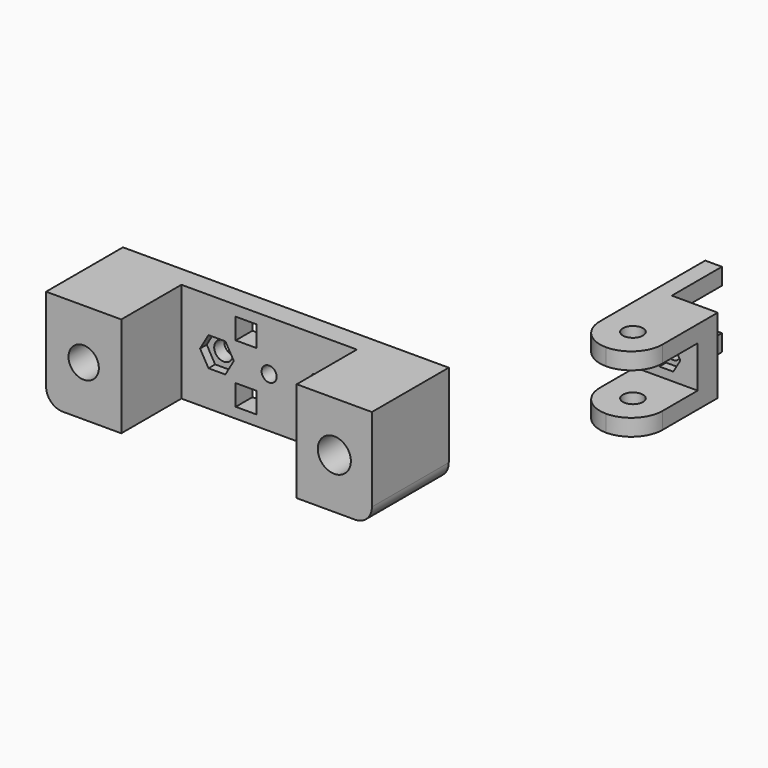
from build123d import *

# Parameters (mm, degrees)
F0_W      = 78
F0_H      = 24
F1_DEPTH  = 5
F2_R      = 2.25
F3_DEPTH  = 25
F4_DEPTH  = 2
F5_W      = 5
F5_H      = 5
F6_DEPTH  = 25
F7_W      = 18
F7_H      = 24
F8_DEPTH  = 18
F9_R      = 3.6317619329
F9_R_2    = 3.9628945372
F10_DEPTH = 30
F11_R     = 4
F2_R_2    = 1.8
F12_DEPTH = 25
F14_DEPTH = 18
F15_W     = 15
F15_H     = 10
F16_DEPTH = 25
F17_W     = 18
F17_H     = 10
F18_DEPTH = 25
F19_R     = 2.4
F20_DEPTH = 25
F21_R     = 7.49999
F22_R     = 1.8
F23_DEPTH = 25
F24_DEPTH = 2


# Not quite as in the source:
# - a fillet or chamfer is up to 0.001 mm smaller than in the source, because OpenCascade refuses the exact size


with BuildPart() as f1:
    # F0 (on Front) → F1 (new body)
    with BuildSketch(Plane.XZ):
        with Locations((-10.7673791122, -2.1172289916)):
            Rectangle(F0_W, F0_H)
    extrude(amount=F1_DEPTH)

    # F2 (on face) → F3 (cut)
    with BuildSketch(Plane.XZ.offset(5)):
        with Locations((-23.2673791122, -2.1172289916)):
            Circle(F2_R)
        with Locations((1.7326208878, -2.1172289916)):
            Circle(F2_R)
    extrude(amount=-F3_DEPTH, mode=Mode.SUBTRACT)

    # F2 (on face) → F4 (cut)
    with BuildSketch(Plane.XZ.offset(5)):
        Polygon((-21.24665317, 1.3827710084), (-25.2881050544, 1.3827710084), (-27.3088309965, -2.1172289916), (-25.2881050544, -5.6172289916), (-21.24665317, -5.6172289916), (-19.2259272279, -2.1172289916), align=None)
        with Locations((-23.2673791122, -2.1172289916)):
            Circle(F2_R, mode=Mode.SUBTRACT)
        Polygon((3.75334683, 1.3827710084), (-0.2881050544, 1.3827710084), (-2.3088309965, -2.1172289916), (-0.2881050544, -5.6172289916), (3.75334683, -5.6172289916), (5.7740727721, -2.1172289916), align=None)
        with Locations((1.7326208878, -2.1172289916)):
            Circle(F2_R, mode=Mode.SUBTRACT)
    extrude(amount=-F4_DEPTH, mode=Mode.SUBTRACT)

    # F5 (on face) → F6 (cut)
    with BuildSketch(Plane.XZ.offset(5)):
        with Locations((-16.2673791122, -9.1172289916)):
            Rectangle(F5_W, F5_H)
        with Locations((-16.2673791122, 4.8827710084)):
            Rectangle(F5_W, F5_H)
    extrude(amount=-F6_DEPTH, mode=Mode.SUBTRACT)

    # F7 (on face) → F8 (join)
    with BuildSketch(Plane.XZ.offset(5)):
        with Locations((-40.7673791122, -2.1172289916)):
            Rectangle(F7_W, F7_H)
        with Locations((19.2326208878, -2.1172289916)):
            Rectangle(F7_W, F7_H)
    extrude(amount=F8_DEPTH)

    # F9 (on face) → F10 (cut, symmetric)
    with BuildSketch(Plane.XZ.offset(5)):
        with Locations((-40.7673791122, -2.1172289916)):
            Circle(F9_R)
        with Locations((19.2326208878, -2.1172289916)):
            Circle(F9_R_2)
    extrude(amount=F10_DEPTH, both=True, mode=Mode.SUBTRACT)

    # F11
    f11_edges = [f1.edges().sort_by_distance(p)[0] for p in [
        (-49.767379, -11.5, -14.117229),
        (28.232621, -11.5, -14.117229),
    ]]
    fillet(f11_edges, radius=F11_R)

    # F2 (on face) → F12 (cut)
    with BuildSketch(Plane.XZ.offset(5)):
        with Locations((-10.7673791122, -2.1172289916)):
            Circle(F2_R_2)
    extrude(amount=-F12_DEPTH, mode=Mode.SUBTRACT)


with BuildPart() as f14:
    # F13 (on Top) → F14 (new body)
    with BuildSketch(Plane.XY):
        Polygon((52.3174511414, 51.6376284141), (48.3174511414, 51.6376284141), (48.3174511414, 12.6376284141), (63.3174511414, 12.6376284141), (63.3174511414, 36.6376284141), (52.3174511414, 36.6376284141), align=None)
    extrude(amount=F14_DEPTH)

    # F15 (on face) → F16 (cut)
    with BuildSketch(Plane.YZ.offset(52.3174511414)):
        with Locations((44.1376284141, 9)):
            Rectangle(F15_W, F15_H)
    extrude(amount=-F16_DEPTH, mode=Mode.SUBTRACT)

    # F17 (on face) → F18 (cut)
    with BuildSketch(Plane.YZ.offset(63.3174511414)):
        with Locations((21.6376284141, 9)):
            Rectangle(F17_W, F17_H)
    extrude(amount=-F18_DEPTH, mode=Mode.SUBTRACT)

    # F19 (on face) → F20 (cut)
    with BuildSketch(Plane.XY.offset(18)):
        with Locations((55.8174511414, 20.6376284141)):
            Circle(F19_R)
    extrude(amount=-F20_DEPTH, mode=Mode.SUBTRACT)

    # F21 (radius 7.5 in the source; OpenCascade refuses exactly that, so slightly less here)
    f21_edges = [f14.edges().sort_by_distance(p)[0] for p in [
        (48.317451, 12.637628, 16),
        (48.317451, 12.637628, 2),
        (63.317451, 12.637628, 2),
        (63.317451, 12.637628, 16),
    ]]
    fillet(f21_edges, radius=F21_R)

    # F22 (on face) → F23 (cut)
    with BuildSketch(Plane.XZ.offset(-30.6376284141)):
        with Locations((55.8174511414, 9)):
            Circle(F22_R)
    extrude(amount=-F23_DEPTH, mode=Mode.SUBTRACT)

    # F22 (on face) → F24 (cut)
    with BuildSketch(Plane.XZ.offset(-30.6376284141)):
        Polygon((57.491766922, 11.9), (54.1431353607, 11.9), (52.4688195801, 9), (54.1431353607, 6.1), (57.491766922, 6.1), (59.1660827027, 9), align=None)
        with Locations((55.8174511414, 9)):
            Circle(F22_R, mode=Mode.SUBTRACT)
    extrude(amount=-F24_DEPTH, mode=Mode.SUBTRACT)


solid = Compound([f1.part, f14.part])
